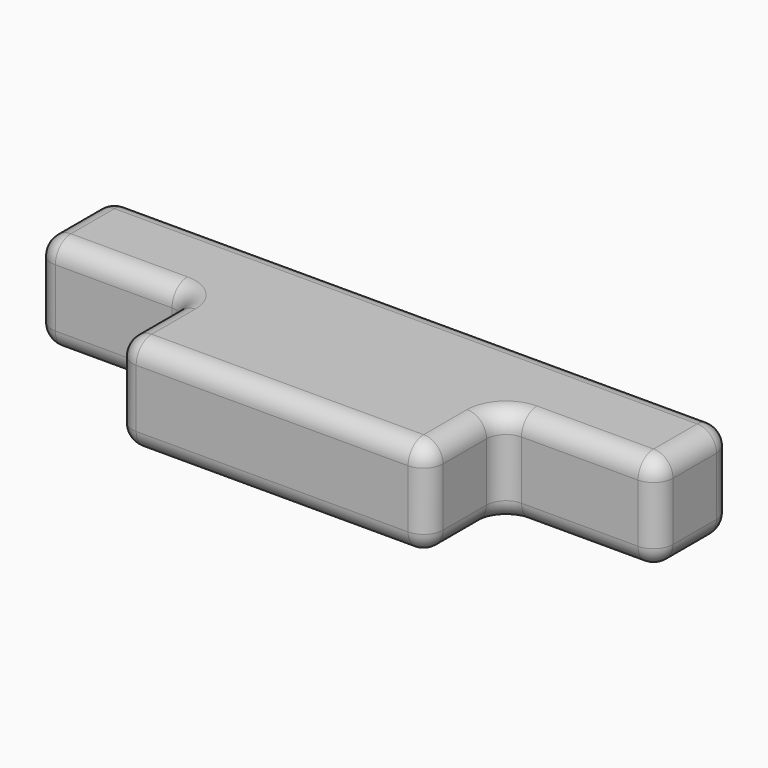
from build123d import *

# Parameters (mm, degrees)
F1_DEPTH = 25
F2_F1_R  = 5
F2_F2_R  = 5


with BuildPart() as f1:
    # F0 (on Top) → F1 (new body)
    with BuildSketch(Plane.XY):
        Polygon((0, 50.3999988563), (-80, 50.3999988563), (-80, 26.3999988563), (-40, 26.3999988563), (-40, 2.3999988563), (40, 2.3999988563), (40, 26.3999988563), (80, 26.3999988563), (80, 50.3999988563), align=None)
    extrude(amount=F1_DEPTH)

    # F2: fillet of radius 5 on 23 edges, made by hand

    # F2_f1
    f2_f1_edges = [f1.edges().sort_by_distance(p)[0] for p in [
        (40, 26.3999988563, 12.5),
        (-40, 26.3999988563, 12.5),
    ]]
    fillet(f2_f1_edges, radius=F2_F1_R)

    # F2_f2
    f2_f2_edges = [f1.edges().sort_by_distance(p)[0] for p in [
        (0, 2.3999988563, 25),
        (-40, 11.8999988563, 25),
        (0, 50.3999988563, 25),
        (-80, 38.3999988563, 25),
        (-62.5, 26.3999988563, 25),
        (40, 11.8999988563, 25),
        (62.5, 26.3999988563, 25),
        (80, 38.3999988563, 25),
        (40, 2.3999988563, 12.5),
        (0, 2.3999988563, 0),
        (40, 11.8999988563, 0),
        (62.5, 26.3999988563, 0),
        (80, 26.3999988563, 12.5),
        (80, 38.3999988563, 0),
        (80, 50.3999988563, 12.5),
        (-40, 2.3999988563, 12.5),
        (-80, 26.3999988563, 12.5),
        (-62.5, 26.3999988563, 0),
        (-80, 50.3999988563, 12.5),
        (-80, 38.3999988563, 0),
        (0, 50.3999988563, 0),
        (-41.4644660941, 24.9355327622, 0),
        (41.4644660941, 24.9355327622, 0),
        (41.4644660941, 24.9355327622, 25),
        (-41.4644660941, 24.9355327622, 25),
    ]]
    fillet(f2_f2_edges, radius=F2_F2_R)


solid = f1.part
